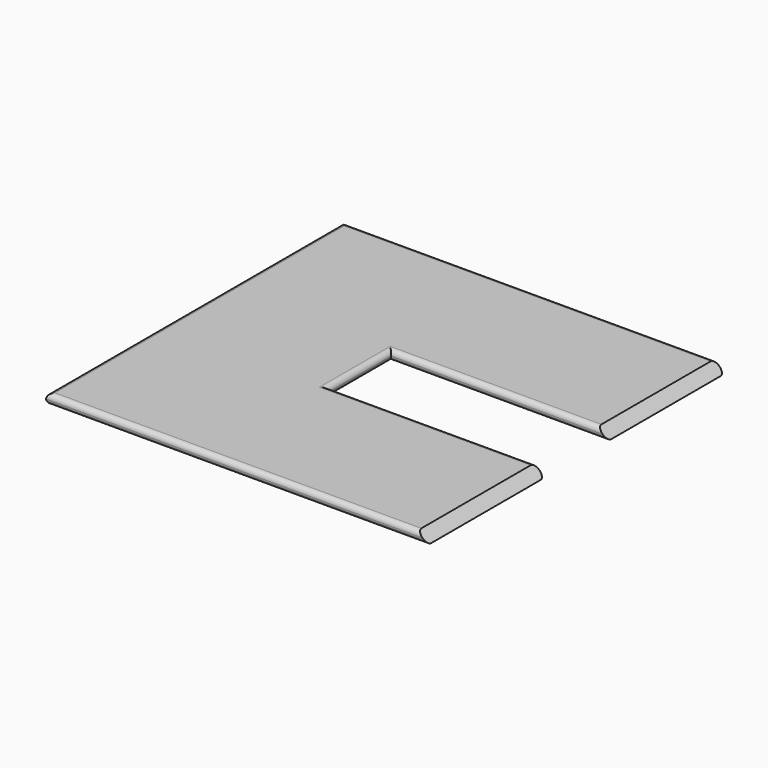
from build123d import *

# Parameters (mm, degrees)
F1_DEPTH     = 5
F2_SIZE      = 4.99999
F3_T1_DEPTH  = 40
F3_T3_DEPTH  = 111.25001
F3_T5_DEPTH  = 12.50001
F3_T7_DEPTH  = 116.25
F3_T9_DEPTH  = 206.5
F3_T11_DEPTH = 201.5
F3_T13_DEPTH = 201.50001
F3_T19_DEPTH = 117.50001
F3_T23_DEPTH = 46.25
F3_T30_DEPTH = 46.25
F3_T34_DEPTH = 117.50001
F3_T41_DEPTH = 122.5
F3_T45_DEPTH = 46.25
F3_T52_DEPTH = 46.25
F3_T56_DEPTH = 122.5


# Not quite as in the source:
# - a fillet or chamfer that OpenCascade refuses, or shapes differently, is made with other operations: its cross-section is extruded or revolved along the edge and cut away or added
# - a fillet or chamfer is up to 0.001 mm smaller than in the source, because OpenCascade refuses the exact size


with BuildPart() as f1:
    # F0 (on Top) → F1 (new body)
    with BuildSketch(Plane.XY):
        Polygon((-97, -94.5), (97, -94.5), (97, -20), (-13, -20), (-13, 20), (97, 20), (97, 94.5), (-97, 94.5), align=None)
    extrude(amount=F1_DEPTH)

    # F2 (size 5 in the source; OpenCascade refuses exactly that, so slightly less here)
    f2_edges = [f1.edges().sort_by_distance(p)[0] for p in [
        (97, -57.25, 5),
        (97, 57.25, 5),
    ]]
    chamfer(f2_edges, length=F2_SIZE)

    # F3: fillet of radius 2.5 on 14 edges, made by hand

    # F3_s2 → F3_t1 (cut)
    with BuildSketch(Plane.XZ.offset(-20)):
        with BuildLine():
            ThreePointArc((-15.5, 5), (-13.732233047, 4.267766953), (-13, 2.5))
            Line((-13, 2.5), (-13, 5))
            Line((-13, 5), (-15.5, 5))
        make_face()
        with BuildLine():
            ThreePointArc((-15.5, 0), (-13.732233047, 0.732233047), (-13, 2.5))
            Line((-13, 2.5), (-13, 0))
            Line((-13, 0), (-15.5, 0))
        make_face()
    extrude(amount=F3_T1_DEPTH, mode=Mode.SUBTRACT)

    # F3_s4 → F3_t3 (cut)
    with BuildSketch(Plane.YZ.offset(-13)):
        with BuildLine():
            ThreePointArc((22.5, 5), (20.732233047, 4.267766953), (20, 2.5))
            Line((20, 2.5), (20, 5))
            Line((20, 5), (22.5, 5))
        make_face()
        with BuildLine():
            ThreePointArc((-22.5, 5), (-20.732233047, 4.267766953), (-20, 2.5))
            Line((-20, 2.5), (-20, 5))
            Line((-20, 5), (-22.5, 5))
        make_face()
    extrude(amount=F3_T3_DEPTH, mode=Mode.SUBTRACT)

    # F3_s6 → F3_t5 (cut)
    with BuildSketch(Plane.XY.offset(-6.25)):
        with BuildLine():
            ThreePointArc((97, -22.5), (96.267766953, -20.732233047), (94.5, -20))
            Line((94.5, -20), (97, -20))
            Line((97, -20), (97, -22.5))
        make_face()
        with BuildLine():
            ThreePointArc((94.5, 20), (96.267766953, 20.732233047), (97, 22.5))
            Line((97, 22.5), (97, 20))
            Line((97, 20), (94.5, 20))
        make_face()
    extrude(amount=F3_T5_DEPTH, mode=Mode.SUBTRACT)

    # F3_s8 → F3_t7 (cut)
    with BuildSketch(Plane.YZ.offset(-13)):
        with BuildLine():
            ThreePointArc((-22.5, 0), (-20.732233047, 0.732233047), (-20, 2.5))
            Line((-20, 2.5), (-20, 0))
            Line((-20, 0), (-22.5, 0))
        make_face()
        with BuildLine():
            ThreePointArc((22.5, 0), (20.732233047, 0.732233047), (20, 2.5))
            Line((20, 2.5), (20, 0))
            Line((20, 0), (22.5, 0))
        make_face()
    extrude(amount=F3_T7_DEPTH, mode=Mode.SUBTRACT)

    # F3_s10 → F3_t9 (cut)
    with BuildSketch(Plane.YZ.offset(-103.25)):
        with BuildLine():
            ThreePointArc((-94.5, 2.5), (-93.767766953, 0.732233047), (-92, 0))
            Line((-92, 0), (-94.5, 0))
            Line((-94.5, 0), (-94.5, 2.5))
        make_face()
        with BuildLine():
            ThreePointArc((92, 0), (93.767766953, 0.732233047), (94.5, 2.5))
            Line((94.5, 2.5), (94.5, 0))
            Line((94.5, 0), (92, 0))
        make_face()
    extrude(amount=F3_T9_DEPTH, mode=Mode.SUBTRACT)

    # F3_s12 → F3_t11 (cut)
    with BuildSketch(Plane.XZ.offset(-100.75)):
        with BuildLine():
            ThreePointArc((-94.5, 0), (-96.267766953, 0.732233047), (-97, 2.5))
            Line((-97, 2.5), (-97, 0))
            Line((-97, 0), (-94.5, 0))
        make_face()
        with BuildLine():
            ThreePointArc((-94.5, 5), (-96.267766953, 4.267766953), (-97, 2.5))
            Line((-97, 2.5), (-97, 5))
            Line((-97, 5), (-94.5, 5))
        make_face()
    extrude(amount=F3_T11_DEPTH, mode=Mode.SUBTRACT)

    # F3_s14 → F3_t13 (cut)
    with BuildSketch(Plane.YZ.offset(-103.25)):
        with BuildLine():
            ThreePointArc((92, 5), (93.767766953, 4.267766953), (94.5, 2.5))
            Line((94.5, 2.5), (94.5, 5))
            Line((94.5, 5), (92, 5))
        make_face()
        with BuildLine():
            ThreePointArc((-94.5, 2.5), (-93.767766953, 4.267766953), (-92, 5))
            Line((-92, 5), (-94.5, 5))
            Line((-94.5, 5), (-94.5, 2.5))
        make_face()
    extrude(amount=F3_T13_DEPTH, mode=Mode.SUBTRACT)


with BuildPart() as f3_tool17:
    # F3_s18 → F3_t19 (new body)
    with BuildSketch(Plane.YZ.offset(98.25001)):
        with BuildLine():
            ThreePointArc((-22.5, 5), (-20.732233047, 4.267766953), (-20, 2.5))
            Line((-20, 2.5), (-20, 5))
            Line((-20, 5), (-22.5, 5))
        make_face()
    extrude(amount=-F3_T19_DEPTH)

    split(bisect_by=Plane.YZ.offset(-13), keep=Keep.BOTTOM)


with BuildPart() as f3_tool21:
    # F3_s22 → F3_t23 (new body)
    with BuildSketch(Plane.XZ.offset(26.25)):
        with BuildLine():
            ThreePointArc((-15.5, 5), (-13.732233047, 4.267766953), (-13, 2.5))
            Line((-13, 2.5), (-13, 5))
            Line((-13, 5), (-15.5, 5))
        make_face()
    extrude(amount=-F3_T23_DEPTH)

    split(bisect_by=Plane.XZ.offset(20), keep=Keep.TOP)


with BuildPart() as f3_tool17_1:
    add(f3_tool17.part)

    # F3_t25: intersect F3_tool21
    add(f3_tool21.part, mode=Mode.INTERSECT)


with BuildPart() as f1_1:
    add(f1.part)

    # F3_t15: cut F3_tool17
    add(f3_tool17_1.part, mode=Mode.SUBTRACT)


with BuildPart() as f3_tool28:
    # F3_s29 → F3_t30 (new body)
    with BuildSketch(Plane.XZ.offset(20)):
        with BuildLine():
            ThreePointArc((-15.5, 5), (-13.732233047, 4.267766953), (-13, 2.5))
            Line((-13, 2.5), (-13, 5))
            Line((-13, 5), (-15.5, 5))
        make_face()
    extrude(amount=-F3_T30_DEPTH)

    split(bisect_by=Plane.XZ.offset(-20), keep=Keep.BOTTOM)


with BuildPart() as f3_tool32:
    # F3_s33 → F3_t34 (new body)
    with BuildSketch(Plane.YZ.offset(-19.25)):
        with BuildLine():
            ThreePointArc((22.5, 5), (20.732233047, 4.267766953), (20, 2.5))
            Line((20, 2.5), (20, 5))
            Line((20, 5), (22.5, 5))
        make_face()
    extrude(amount=F3_T34_DEPTH)

    split(bisect_by=Plane.YZ.offset(-13), keep=Keep.BOTTOM)


with BuildPart() as f3_tool28_1:
    add(f3_tool28.part)

    # F3_t36: intersect F3_tool32
    add(f3_tool32.part, mode=Mode.INTERSECT)


with BuildPart() as f1_2:
    add(f1_1.part)

    # F3_t26: cut F3_tool28
    add(f3_tool28_1.part, mode=Mode.SUBTRACT)


with BuildPart() as f3_tool39:
    # F3_s40 → F3_t41 (new body)
    with BuildSketch(Plane.YZ.offset(103.25)):
        with BuildLine():
            ThreePointArc((-22.5, 0), (-20.732233047, 0.732233047), (-20, 2.5))
            Line((-20, 2.5), (-20, 0))
            Line((-20, 0), (-22.5, 0))
        make_face()
    extrude(amount=-F3_T41_DEPTH)

    split(bisect_by=Plane.YZ.offset(-13), keep=Keep.BOTTOM)


with BuildPart() as f3_tool43:
    # F3_s44 → F3_t45 (new body)
    with BuildSketch(Plane.XZ.offset(26.25)):
        with BuildLine():
            ThreePointArc((-15.5, 0), (-13.732233047, 0.732233047), (-13, 2.5))
            Line((-13, 2.5), (-13, 0))
            Line((-13, 0), (-15.5, 0))
        make_face()
    extrude(amount=-F3_T45_DEPTH)

    split(bisect_by=Plane.XZ.offset(20), keep=Keep.TOP)


with BuildPart() as f3_tool39_1:
    add(f3_tool39.part)

    # F3_t47: intersect F3_tool43
    add(f3_tool43.part, mode=Mode.INTERSECT)


with BuildPart() as f1_3:
    add(f1_2.part)

    # F3_t37: cut F3_tool39
    add(f3_tool39_1.part, mode=Mode.SUBTRACT)


with BuildPart() as f3_tool50:
    # F3_s51 → F3_t52 (new body)
    with BuildSketch(Plane.XZ.offset(20)):
        with BuildLine():
            ThreePointArc((-15.5, 0), (-13.732233047, 0.732233047), (-13, 2.5))
            Line((-13, 2.5), (-13, 0))
            Line((-13, 0), (-15.5, 0))
        make_face()
    extrude(amount=-F3_T52_DEPTH)

    split(bisect_by=Plane.XZ.offset(-20), keep=Keep.BOTTOM)


with BuildPart() as f3_tool54:
    # F3_s55 → F3_t56 (new body)
    with BuildSketch(Plane.YZ.offset(-19.25)):
        with BuildLine():
            ThreePointArc((22.5, 0), (20.732233047, 0.732233047), (20, 2.5))
            Line((20, 2.5), (20, 0))
            Line((20, 0), (22.5, 0))
        make_face()
    extrude(amount=F3_T56_DEPTH)

    split(bisect_by=Plane.YZ.offset(-13), keep=Keep.BOTTOM)


with BuildPart() as f3_tool50_1:
    add(f3_tool50.part)

    # F3_t58: intersect F3_tool54
    add(f3_tool54.part, mode=Mode.INTERSECT)


with BuildPart() as f1_4:
    add(f1_3.part)

    # F3_t48: cut F3_tool50
    add(f3_tool50_1.part, mode=Mode.SUBTRACT)


solid = f1_4.part
